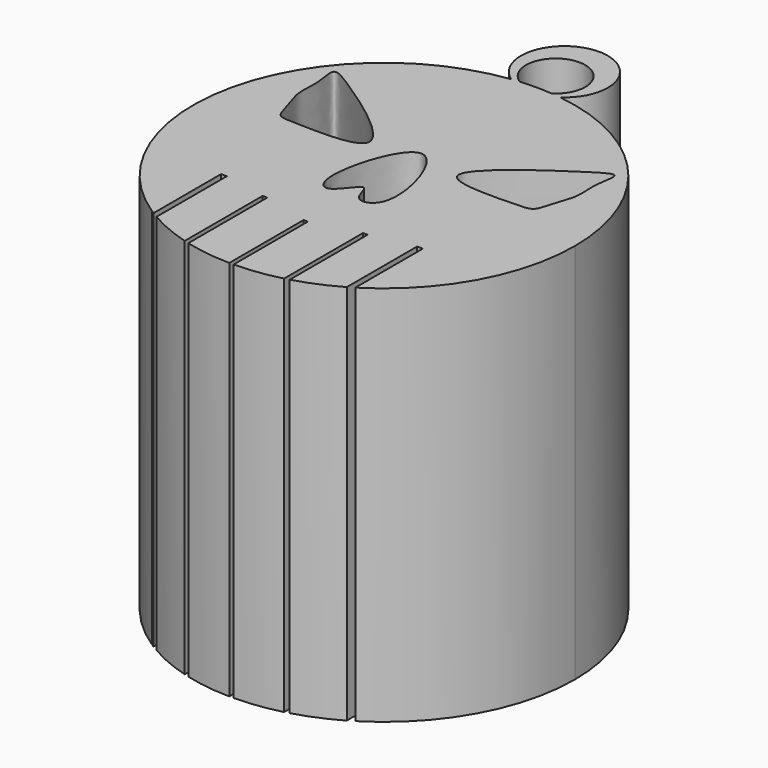
from build123d import *

# Parameters (mm, degrees)
F1_DEPTH = 25.4


with BuildPart() as f1:
    # F0 (on Top) → F1 (new body)
    with BuildSketch(Plane.XY):
        with BuildLine():
            ThreePointArc((6.7156300194, -0.961144645), (11.103569274, 3.653541643), (12.7, 9.8180164282))
            ThreePointArc((12.7, 9.8180164282), (9.5449480524, 18.1956035913), (1.6474068226, 22.4107147395))
            ThreePointArc((1.6474068226, 22.4107147395), (1.3388234894, 22.4472504376), (1.0294386506, 22.4762254667))
            ThreePointArc((1.0294386506, 22.4762254667), (-0.028773145, 22.5179838339), (-1.086784862, 22.4714309343))
            ThreePointArc((-1.086784862, 22.4714309343), (-1.3485915697, 22.4462111043), (-1.6098198538, 22.4155749233))
            ThreePointArc((-1.6098198538, 22.4155749233), (-12.3800103209, 12.6509203191), (-6.9281209855, -0.8258146307))
            Line((-6.9281209855, -0.8258146307), (-6.8822319383, -0.8258146307))
            Line((-6.8822319383, -0.8258146307), (-6.8822319383, -0.855543594))
            ThreePointArc((-6.8822319383, -0.855543594), (-6.7991360003, -0.9086675725), (-6.7156300194, -0.961144645))
            Line((-6.7156300194, -0.961144645), (-6.7156300194, 4.6587398687))
            Line((-6.7156300194, 4.6587398687), (-6.3310727347, 4.6587398687))
            Line((-6.3310727347, 4.6587398687), (-6.3310727347, -1.1914121687))
            ThreePointArc((-6.3310727347, -1.1914121687), (-4.9495356332, -1.8777989353), (-3.4949700482, -2.3916184706))
            Line((-3.4949700482, -2.3916184706), (-3.4949700482, 4.0883066069))
            Line((-3.4949700482, 4.0883066069), (-3.1876309074, 4.0883066069))
            Line((-3.1876309074, 4.0883066069), (-3.1876309074, -2.4754374884))
            ThreePointArc((-3.1876309074, -2.4754374884), (-1.6746684307, -2.7710854321), (-0.13703122, -2.8812442765))
            Line((-0.13703122, -2.8812442765), (-0.13703122, 3.3066231491))
            Line((-0.13703122, 3.3066231491), (0.1494322853, 3.3066231491))
            Line((0.1494322853, 3.3066231491), (0.1494322853, -2.8811044072))
            ThreePointArc((0.1494322853, -2.8811044072), (1.6808150107, -2.7702662546), (3.1876309074, -2.4754374884))
            Line((3.1876309074, -2.4754374884), (3.1876309074, 4.0883066069))
            Line((3.1876309074, 4.0883066069), (3.4949700482, 4.0883066069))
            Line((3.4949700482, 4.0883066069), (3.4949700482, -2.3916184706))
            ThreePointArc((3.4949700482, -2.3916184706), (4.9495356332, -1.8777989353), (6.3310727347, -1.1914121687))
            Line((6.3310727347, -1.1914121687), (6.3310727347, 4.6587398687))
            Line((6.3310727347, 4.6587398687), (6.7156300194, 4.6587398687))
            Line((6.7156300194, 4.6587398687), (6.7156300194, -0.961144645))
        make_face()
        with BuildLine():
            add(Edge.make_bspline(
                [(0, 12.9685981976), (-1.1262707569, 13.0608157796), (-2.748365158, 7.936569366), (-1.2735758817, 6.2577367621), (0.1843082925, 8.9908750032), (0.2962277728, 6.5228781858), (2.9280933099, 7.2517179831), (1.1483668305, 12.8745714179), (0, 12.9685981976)],
                knots=[0, 0, 0, 0, 0.2461617493, 0.3674777738, 0.5071240723, 0.6245056694, 0.7490088542, 1, 1, 1, 1], degree=3))
        make_face(mode=Mode.SUBTRACT)
        with BuildLine():
            add(Edge.make_bspline(
                [(-8.0023061995, 16.7331782252), (-6.2510557676, 15.6142079944), (0.0505703268, 11.3072332803), (-7.1931373209, 11.5741872719), (-8.536675253, 11.5601551472), (-8.7321601562, 12.6489403605), (-9.4405060529, 14.3126079871), (-9.1067828933, 15.7231243812), (-9.6696121761, 17.7306750622), (-8.8186828026, 17.2548061427), (-8.0023061995, 16.7331782252)],
                knots=[0, 0, 0, 0, 0.2214766404, 0.3948821826, 0.4949979166, 0.5749687847, 0.6880101274, 0.7951541475, 0.8967547165, 1, 1, 1, 1], degree=3))
        make_face(mode=Mode.SUBTRACT)
        with BuildLine():
            add(Edge.make_bspline(
                [(8.0023061995, 16.7331782252), (6.2510557676, 15.6142079944), (-0.0505703268, 11.3072332803), (7.1931373209, 11.5741872719), (8.536675253, 11.5601551472), (8.7321601562, 12.6489403605), (9.4405060529, 14.3126079871), (9.1067828933, 15.7231243812), (9.6696121761, 17.7306750622), (8.8186828026, 17.2548061427), (8.0023061995, 16.7331782252)],
                knots=[0, 0, 0, 0, 0.2214766404, 0.3948821826, 0.4949979166, 0.5749687847, 0.6880101274, 0.7951541475, 0.8967547165, 1, 1, 1, 1], degree=3))
        make_face(mode=Mode.SUBTRACT)
        with BuildLine():
            ThreePointArc((1.0294386506, 22.4762254667), (1.3388234894, 22.4472504376), (1.6474068226, 22.4107147395))
            ThreePointArc((1.6474068226, 22.4107147395), (0.0266660272, 27.6892120738), (-1.6098198538, 22.4155749233))
            ThreePointArc((-1.6098198538, 22.4155749233), (-1.3485915697, 22.4462111043), (-1.086784862, 22.4714309343))
            ThreePointArc((-1.086784862, 22.4714309343), (-0.0369259735, 26.1165009701), (1.0294386506, 22.4762254667))
        make_face()
    extrude(amount=F1_DEPTH)


solid = f1.part
